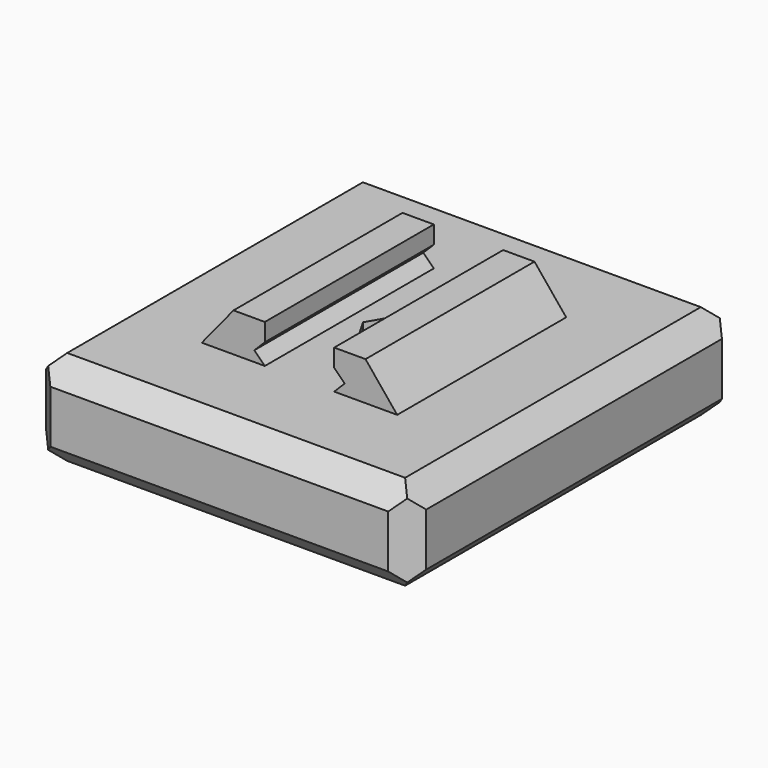
from build123d import *

# Parameters (mm, degrees)
F0_W       = 91.4399989891
F0_H       = 99.0599989891
F0_W_2     = 81.28
F0_H_2     = 88.9
F1_DEPTH   = 17.78
F2_W       = 91.4399989891
F2_H       = 99.0599989891
F3_DEPTH   = 5.08
F4_SIZE    = 5.08
F6_DEPTH   = 25.4
F7_R       = 2.286
F8_DEPTH   = 25.4
F10_DEPTH  = 2.54
F11_SIZE   = 5.07999
F11_SIZE_2 = 5.08
F13_DEPTH  = 50.8


# Not quite as in the source:
# - a fillet or chamfer is up to 0.001 mm smaller than in the source, because OpenCascade refuses the exact size


with BuildPart() as f1:
    # F0 (on Top) → F1 (new body)
    with BuildSketch(Plane.XY):
        Rectangle(F0_W, F0_H)
        Rectangle(F0_W_2, F0_H_2, mode=Mode.SUBTRACT)
    extrude(amount=-F1_DEPTH)

    # F2 (on face) → F3 (join)
    with BuildSketch(Plane.XY):
        Rectangle(F2_W, F2_H)
    extrude(amount=F3_DEPTH)

    # F4
    f4_edges = [f1.edges().sort_by_distance(p)[0] for p in [
        (-45.719999, 49.529999, -6.35),
        (45.719999, 49.529999, -6.35),
        (45.719999, -49.529999, -6.35),
        (-45.719999, -49.529999, -6.35),
    ]]
    chamfer(f4_edges, length=F4_SIZE)

    # F5 (on Front) → F6 (join, symmetric)
    with BuildSketch(Plane.XZ):
        Polygon((10.8585, 7.5946), (8.3439, 5.08), (15.875, 5.08), (15.875, 14.4018), (8.3439, 14.4018), (8.3439, 10.1092), align=None)
        Polygon((-8.3439, 10.1092), (-8.3439, 14.4018), (-15.875, 14.4018), (-15.875, 5.08), (-8.3439, 5.08), (-10.8585, 7.5946), align=None)
    extrude(amount=F6_DEPTH, both=True)

    # F7 (on face) → F8 (cut)
    with BuildSketch(Plane(origin=(0, 0, 0), x_dir=(1, 0, 0), z_dir=(0, 0, -1))):
        Circle(F7_R)
    extrude(amount=-F8_DEPTH, mode=Mode.SUBTRACT)

    # F9 (on face) → F10 (cut)
    with BuildSketch(Plane.XY.offset(5.08)):
        Polygon((2.5204947689, 4.365625), (-2.5204947689, 4.365625), (-5.0409895379, 0), (-2.5204947689, -4.365625), (2.5204947689, -4.365625), (5.0409895379, 0), align=None)
    extrude(amount=-F10_DEPTH, mode=Mode.SUBTRACT)

    # F11 (call 1 of 8: OpenCascade refuses the feature's edges together) (size 5.08 in the source; OpenCascade refuses exactly that, so slightly less here)
    f11_edges = [f1.edges().sort_by_distance(p)[0] for p in [
        (0, 49.529999, -17.78),
    ]]
    chamfer(f11_edges, length=F11_SIZE)

    # F11#2 (call 2 of 8) (size 5.08 in the source; OpenCascade refuses exactly that, so slightly less here)
    f11_2_edges = [f1.edges().sort_by_distance(p)[0] for p in [
        (-45.719999, 0, -17.78),
    ]]
    chamfer(f11_2_edges, length=F11_SIZE)

    # F11#3 (call 3 of 8) (size 5.08 in the source; OpenCascade refuses exactly that, so slightly less here)
    f11_3_edges = [f1.edges().sort_by_distance(p)[0] for p in [
        (0, -49.529999, -17.78),
    ]]
    chamfer(f11_3_edges, length=F11_SIZE)

    # F11#4 (call 4 of 8) (size 5.08 in the source; OpenCascade refuses exactly that, so slightly less here)
    f11_4_edges = [f1.edges().sort_by_distance(p)[0] for p in [
        (45.719999, 0, -17.78),
    ]]
    chamfer(f11_4_edges, length=F11_SIZE)

    # F11#5 (call 5 of 8)
    f11_5_edges = [f1.edges().sort_by_distance(p)[0] for p in [
        (0, 49.529999, 5.08),
    ]]
    chamfer(f11_5_edges, length=F11_SIZE_2)

    # F11#6 (call 6 of 8)
    f11_6_edges = [f1.edges().sort_by_distance(p)[0] for p in [
        (-45.719999, 0, 5.08),
    ]]
    chamfer(f11_6_edges, length=F11_SIZE_2)

    # F11#7 (call 7 of 8)
    f11_7_edges = [f1.edges().sort_by_distance(p)[0] for p in [
        (0, -49.529999, 5.08),
    ]]
    chamfer(f11_7_edges, length=F11_SIZE_2)

    # F11#8 (call 8 of 8)
    f11_8_edges = [f1.edges().sort_by_distance(p)[0] for p in [
        (45.719999, 0, 5.08),
    ]]
    chamfer(f11_8_edges, length=F11_SIZE_2)

    # F12 (on face) → F13 (join, through all)
    with BuildSketch(Plane.XZ.offset(25.4)):
        Polygon((-15.875, 14.4018), (-23.495, 5.08), (-15.875, 5.08), align=None)
        Polygon((23.495, 5.08), (15.875, 14.4018), (15.875, 5.08), align=None)
    extrude(amount=-F13_DEPTH)


solid = f1.part
